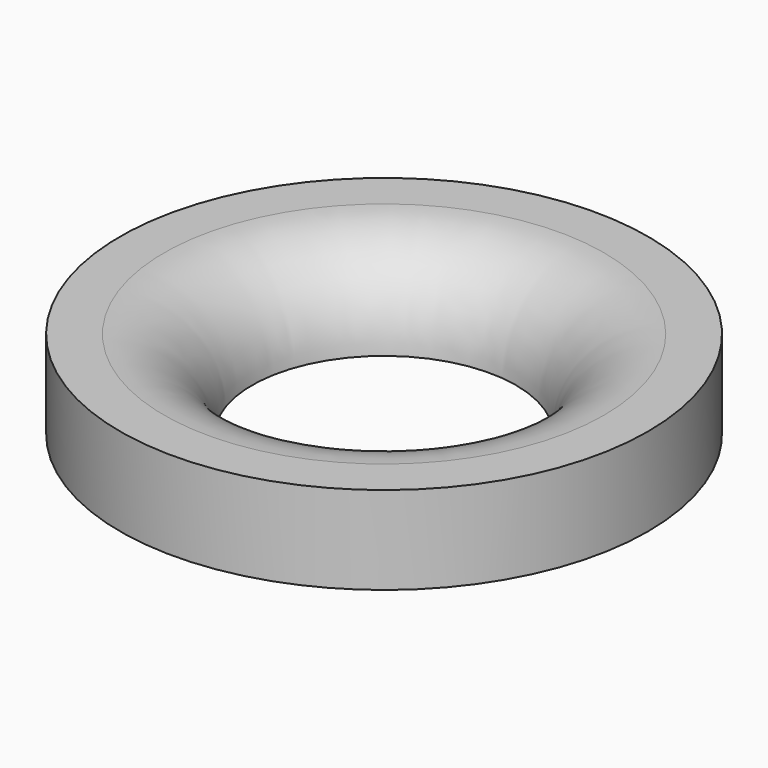
from build123d import *

# Parameters (mm, degrees)
F0_R     = 76.2
F0_R_2   = 38.1
F1_DEPTH = 25.4
F2_R     = 25.39999


# Not quite as in the source:
# - a fillet or chamfer is up to 0.001 mm smaller than in the source, because OpenCascade refuses the exact size


with BuildPart() as f1:
    # F0 (on Top) → F1 (new body)
    with BuildSketch(Plane.XY):
        Circle(F0_R)
        Circle(F0_R_2, mode=Mode.SUBTRACT)
    extrude(amount=F1_DEPTH)

    # F2 (radius 25.4 in the source; OpenCascade refuses exactly that, so slightly less here)
    f2_edges = [f1.edges().sort_by_distance(p)[0] for p in [
        (-38.1, 0, 25.4),
    ]]
    fillet(f2_edges, radius=F2_R)


solid = f1.part
